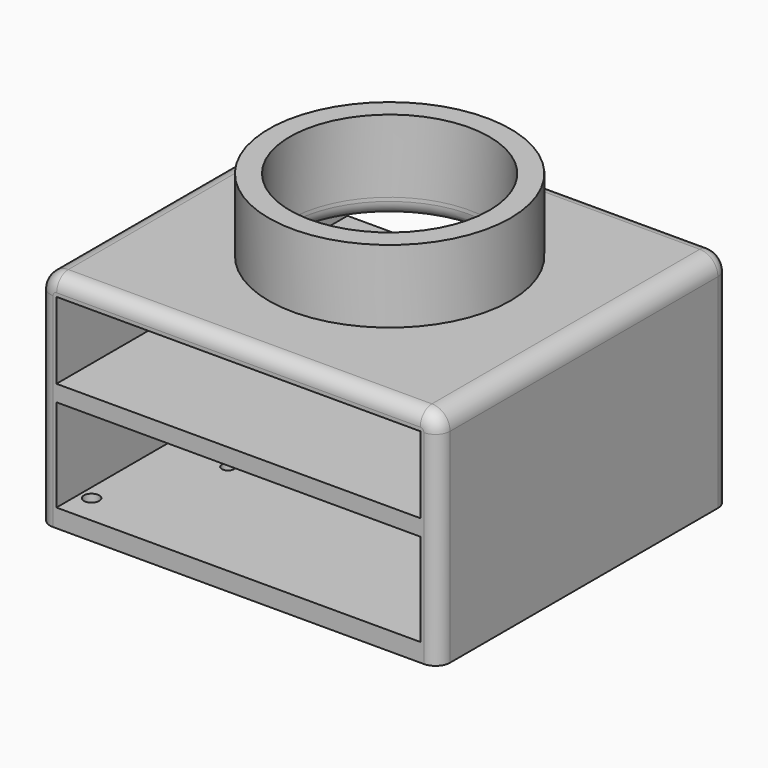
from build123d import *

# Parameters (mm, degrees)
F0_W     = 127
F0_H     = 32.3606841266
F0_H_2   = 26.7147784284
F1_DEPTH = 127
F2_R     = 5.08
F3_R     = 2.1310745611
F4_DEPTH = 25.4
F5_R     = 2.6680723022
F6_DEPTH = 25.4
F7_R     = 42.1805785401
F7_R_2   = 34.8133831429
F8_DEPTH = 25.4
F9_DEPTH = 25.4
F10_R    = 5.08


with BuildPart() as f1:
    # F0 (on Front) → F1 (new body)
    with BuildSketch(Plane.XZ):
        with BuildLine():
            ThreePointArc((69.8099806905, 32.3913091956), (67.950108751, 36.8814372561), (63.4599806905, 38.7413091956))
            Line((63.4599806905, 38.7413091956), (-63.4599806905, 38.7413091956))
            ThreePointArc((-63.4599806905, 38.7413091956), (-67.950108751, 36.8814372561), (-69.8099806905, 32.3913091956))
            Line((-69.8099806905, 32.3913091956), (-69.8099806905, -38.7413091956))
            Line((-69.8099806905, -38.7413091956), (69.8099806905, -38.7413091956))
            Line((69.8099806905, -38.7413091956), (69.8099806905, 32.3913091956))
        make_face()
        with Locations((-0.0400193095, -16.1803420633)):
            Rectangle(F0_W, F0_H, mode=Mode.SUBTRACT)
        with Locations((-0.0400193095, 19.0339199814)):
            Rectangle(F0_W, F0_H_2, mode=Mode.SUBTRACT)
    extrude(amount=F1_DEPTH)

    # F2
    f2_edges = [f1.edges().sort_by_distance(p)[0] for p in [
        (69.809981, -127, -3.175),
        (67.950109, -127, 36.881437),
        (0, -127, 38.741309),
        (-67.950109, -127, 36.881437),
        (-69.809981, -127, -3.175),
        (69.809981, 0, -3.175),
        (67.950109, 0, 36.881437),
        (0, 0, 38.741309),
        (-67.950109, 0, 36.881437),
        (-69.809981, 0, -3.175),
    ]]
    fillet(f2_edges, radius=F2_R)

    # F3 (on face) → F4 (cut)
    with BuildSketch(Plane(origin=(0, 0, -38.7413091956), x_dir=(1, 0, 0), z_dir=(0, 0, -1))):
        with Locations((-42.0244000852, 79.0478363633)):
            Circle(F3_R)
        with Locations((-42.0244000852, 50.4565563633)):
            Circle(F3_R)
        with Locations((39.2230374546, 79.047831549)):
            Circle(F3_R)
        with Locations((39.2230374546, 50.456551549)):
            Circle(F3_R)
    extrude(amount=-F4_DEPTH, mode=Mode.SUBTRACT)

    # F5 (on face) → F6 (cut)
    with BuildSketch(Plane(origin=(0, 0, -38.7413091956), x_dir=(1, 0, 0), z_dir=(0, 0, -1))):
        with Locations((-59.5310516655, 116.688169539)):
            Circle(F5_R)
        with Locations((-59.98695, 10.82233)):
            Circle(F5_R)
        with Locations((58.6440783345, 116.688169539)):
            Circle(F5_R)
        with Locations((58.18818, 10.82233)):
            Circle(F5_R)
    extrude(amount=-F6_DEPTH, mode=Mode.SUBTRACT)

    # F7 (on face) → F8 (join)
    with BuildSketch(Plane.XY.offset(38.7413091956)):
        with Locations((0, -61.0473752022)):
            Circle(F7_R)
        with Locations((0, -61.0473752022)):
            Circle(F7_R_2, mode=Mode.SUBTRACT)
    extrude(amount=F8_DEPTH)

    # F9 (cut): a face of the model
    f9_faces = [f1.faces().sort_by_distance(p)[0] for p in [
        (0, -61.0473752022, 38.7413091956),
    ]]
    extrude(f9_faces, amount=-F9_DEPTH, mode=Mode.SUBTRACT)

    # F10
    f10_edges = [f1.edges().sort_by_distance(p)[0] for p in [
        (-34.813383, -61.047375, 32.391309),
    ]]
    fillet(f10_edges, radius=F10_R)


solid = f1.part
